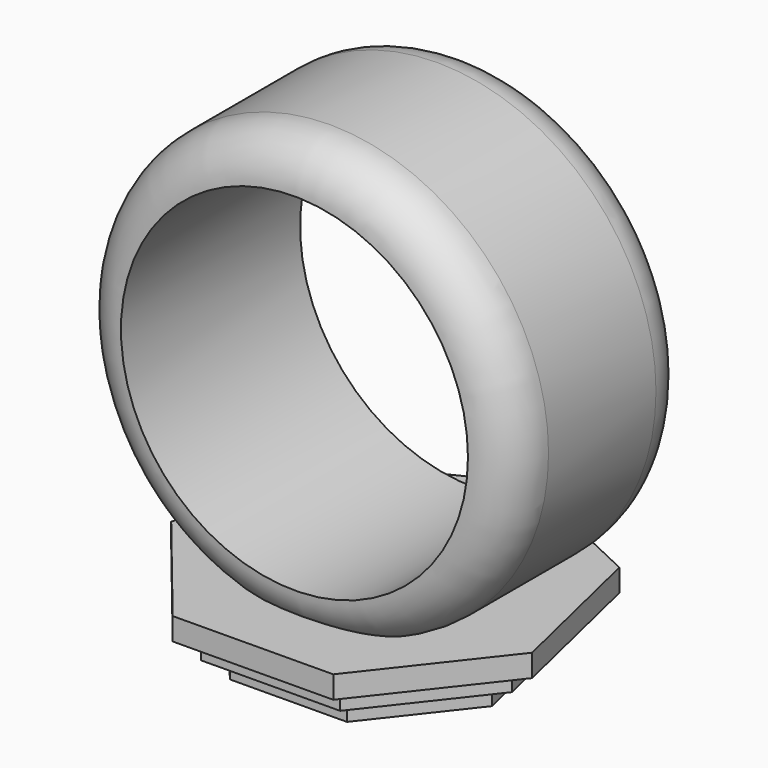
from build123d import *

# Parameters (mm, degrees)
F0_R         = 9.75
F0_R_2       = 7.75
F1_DEPTH     = 5
F2_R         = 1.99999
F4_DEPTH     = 1
F6_DEPTH     = 1
F8_DEPTH     = 1
F9_TEXT_SIZE = 8.3333333333
F10_DEPTH    = 1


# Not quite as in the source:
# - a fillet or chamfer is up to 0.001 mm smaller than in the source, because OpenCascade refuses the exact size
# - Text() gives the source's letters only with a copy of the font that has no kerning and outlines rounded to 1/6400 em; it was checked with that copy


with BuildPart() as f1:
    # F0 (on Front) → F1 (new body, symmetric)
    with BuildSketch(Plane.XZ):
        with Locations((0, 9.9102808163)):
            Circle(F0_R)
        with Locations((0, 9.9102808163)):
            Circle(F0_R_2, mode=Mode.SUBTRACT)
    extrude(amount=F1_DEPTH, both=True)

    # F2 (radius 2 in the source; OpenCascade refuses exactly that, so slightly less here)
    f2_edges = [f1.edges().sort_by_distance(p)[0] for p in [
        (-9.75, -5, 9.910281),
        (-9.75, 5, 9.910281),
    ]]
    fillet(f2_edges, radius=F2_R)


with BuildPart() as f4:
    # F3 (on Top) → F4 (new body)
    with BuildSketch(Plane.XY):
        Polygon((8.0197002668, -1.7575094563), (6.374277554, 5.1742649259), (-0.0711061685, 8.2097122831), (-6.4629454959, 5.0630788436), (-7.9880550448, -1.8961562332), (-3.4979962183, -7.4275469918), (3.6261251066, -7.3658433713), align=None)
    extrude(amount=F4_DEPTH)


with BuildPart() as f6:
    # F5 (on face) → F6 (new body)
    with BuildSketch(Plane(origin=(0, 0, 0), x_dir=(1, 0, 0), z_dir=(0, 0, -1))):
        Polygon((-5.5892170352, -4.3785989749), (-0.0614932941, -7.0998376478), (5.5125361517, -4.4747537616), (6.9355134401, 1.5199109755), (3.1359076494, 6.3700517474), (-3.0251005622, 6.4234136282), (-6.9081463496, 1.6398140332), align=None)
    extrude(amount=F6_DEPTH)


with BuildPart() as f8:
    # F7 (on face) → F8 (new body)
    with BuildSketch(Plane(origin=(0, 0, -1), x_dir=(1, 0, 0), z_dir=(0, 0, -1))):
        Polygon((-2.552204906, 5.4192802647), (-5.8282376544, 1.3834718332), (-4.7154885746, -3.6941191063), (-0.0518804198, -5.9899630125), (4.6507947494, -3.7752425973), (5.8513266133, 1.2823124946), (2.6456901921, 5.3742601236), align=None)
    extrude(amount=F8_DEPTH)


with BuildPart() as f10:
    # F9 (on face) → F10 (new body)
    with BuildSketch(Plane(origin=(0, 0, -2), x_dir=(1, 0, 0), z_dir=(0, 0, -1))):
        with Locations((-3.5579427083, -2.8432416339)):
            Text('ft', F9_TEXT_SIZE, font='Open Sans', font_style=FontStyle.BOLD, text_align=(TextAlign.LEFT, TextAlign.BOTTOM))
    extrude(amount=F10_DEPTH)


solid = Compound([f1.part, f4.part, f6.part, f8.part, f10.part])
